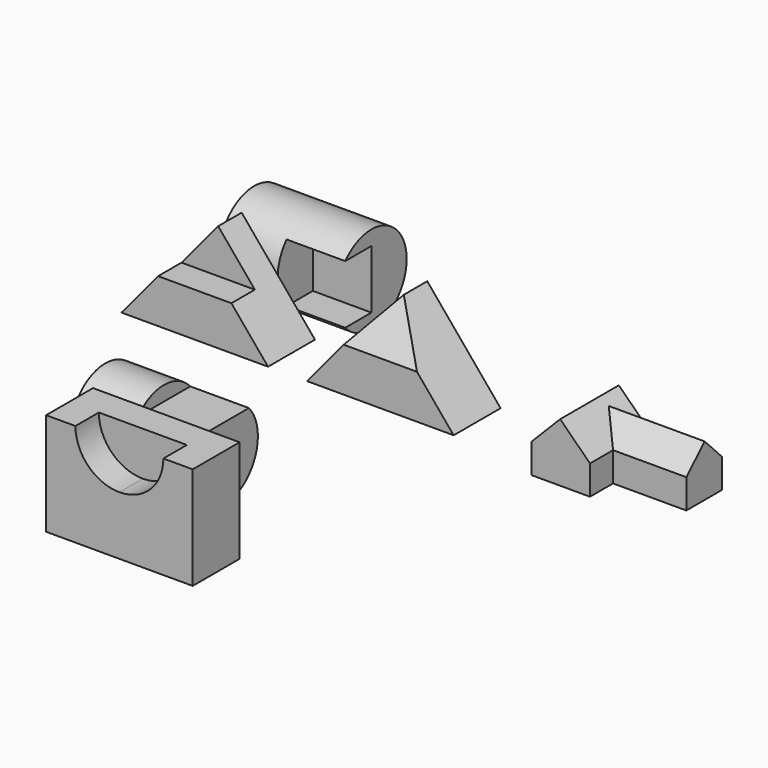
from build123d import *

# Parameters (mm, degrees)
F1_DEPTH  = 101.6
F3_DEPTH  = 50.8
F5_DEPTH  = 50.8
F8_DEPTH  = 254
F10_DEPTH = 101.6
F12_DEPTH = 127
F13_W     = 77.0500511372
F13_H     = 50.8
F14_DEPTH = 127
F17_DEPTH = 203.2
F20_DEPTH = 101.6
F22_DEPTH = 203.2
F24_DEPTH = 101.6
F25_W     = 101.6
F25_H     = 177.8
F26_DEPTH = 254
F28_DEPTH = 50.8


# Not quite as in the source:
# - a feature of the source that left no trace in its solid (it failed there, or was rolled back) is left out


with BuildPart() as f1:
    # F0 (on Front) → F1 (new body)
    with BuildSketch(Plane.XZ):
        Polygon((63.5, 76.2), (0, 0), (254, 0), (190.5, 76.2), align=None)
        Polygon((127, 152.4), (63.5, 76.2), (190.5, 76.2), align=None)
    extrude(amount=F1_DEPTH)

    # F2 (on face) → F3 (join)
    with BuildSketch(Plane.XZ.offset(101.6)):
        Polygon((127, 152.4), (63.5, 76.2), (190.5, 76.2), align=None)
    extrude(amount=-F3_DEPTH)

    # F4 (on face) → F5 (cut)
    with BuildSketch(Plane.XZ.offset(101.6)):
        Polygon((127, 152.4), (63.5, 76.2), (190.5, 76.2), align=None)
    extrude(amount=-F5_DEPTH, mode=Mode.SUBTRACT)


with BuildPart() as f8:
    # F7 (on offset) → F8 (new body)
    with BuildSketch(Plane.YZ.offset(321.564)):
        Polygon((-101.6, 0), (0, 0), (0, 152.4), (-50.8, 152.4), (-101.6, 76.2), align=None)
    extrude(amount=F8_DEPTH)

    # F9 (on face) → F10 (cut)
    with BuildSketch(Plane.XZ.offset(101.6)):
        Polygon((321.564, 76.2), (385.064, 76.2), (448.564, 152.4), (321.564, 152.4), align=None)
        Polygon((321.564, 76.2), (321.564, 0), (385.064, 76.2), align=None)
        Polygon((512.064, 76.2), (575.564, 0), (575.564, 76.2), align=None)
        Polygon((448.564, 152.4), (512.064, 76.2), (575.564, 76.2), (575.564, 152.4), align=None)
    extrude(amount=-F10_DEPTH, mode=Mode.SUBTRACT)


with BuildPart() as f12:
    # F11 (on Front) → F12 (new body)
    with BuildSketch(Plane.XZ):
        Polygon((730.4162154386, 50.8), (730.4162154386, 0), (781.2162154386, 0), (780.4500848747, 101.6), align=None)
        Polygon((780.4500848747, 101.6), (781.2162154386, 0), (832.0162154386, 0), (832.0162154386, 50.8), align=None)
    extrude(amount=F12_DEPTH)

    # F13 (on face) → F14 (join)
    with BuildSketch(Plane.YZ.offset(832.0162154386)):
        Polygon((-77.0500511372, 50.8), (0, 50.8), (-37.422735244, 89.3092527986), align=None)
        with Locations((-38.5250255686, 25.4)):
            Rectangle(F13_W, F13_H)
    extrude(amount=F14_DEPTH)

    # F13 (on face) → F15 (join, up to the next surface of F12)
    with BuildSketch(Plane.YZ.offset(832.0162154386)):
        Polygon((-77.0500511372, 50.8), (0, 50.8), (-37.422735244, 89.3092527986), align=None)
    extrude(until=Until.NEXT, dir=(-1, 0, 0))


with BuildPart() as f17:
    # F16 (on Right) → F17 (new body)
    with BuildSketch(Plane.YZ):
        with BuildLine():
            ThreePointArc((-136.3018900156, -215.5146067858), (-82.4203532892, -193.1961435122), (-60.1018900156, -139.3146067858))
            ThreePointArc((-60.1018900156, -139.3146067858), (-65.0951570451, -112.1845279125), (-79.4205561487, -88.6100324604))
            Line((-79.4205561487, -88.6100324604), (-140.1142077817, -88.6100324604))
            Line((-140.1142077817, -88.6100324604), (-193.1832238825, -88.6100324604))
            ThreePointArc((-193.1832238825, -88.6100324604), (-205.8365165106, -170.4815077899), (-136.3018900156, -215.5146067858))
        make_face()
        with BuildLine():
            Line((-140.1142077817, -88.6100324604), (-79.4205561487, -88.6100324604))
            ThreePointArc((-79.4205561487, -88.6100324604), (-136.3018900156, -63.1146067858), (-193.1832238825, -88.6100324604))
            Line((-193.1832238825, -88.6100324604), (-140.1142077817, -88.6100324604))
        make_face()
    extrude(amount=F17_DEPTH)

    # F18 (on face) → F20 (cut)
    with BuildSketch(Plane.YZ.offset(203.2)):
        with BuildLine():
            Line((-193.0983693738, -88.5150011523), (-136.5470457015, -88.5150011523))
            Line((-136.5470457015, -88.5150011523), (-79.5054106574, -88.5150011523))
            ThreePointArc((-79.5054106574, -88.5150011523), (-136.3018900156, -63.1146067858), (-193.0983693738, -88.5150011523))
        make_face()
    extrude(amount=-F20_DEPTH, mode=Mode.SUBTRACT)


with BuildPart() as f22:
    # F21 (on Right) → F22 (new body)
    with BuildSketch(Plane.YZ):
        with BuildLine():
            ThreePointArc((185.844445633, 76.2), (131.9629089065, -53.8815367264), (262.044445633, 0))
            ThreePointArc((262.044445633, 0), (239.7259823594, 53.8815367264), (185.844445633, 76.2))
        make_face()
    extrude(amount=F22_DEPTH)

    # F23 (on face) → F24 (cut)
    with BuildSketch(Plane.YZ.offset(203.2)):
        with BuildLine():
            ThreePointArc((129.0483190045, 50.8), (114.66051188, 27.1898432407), (109.644445633, 0))
            Line((109.644445633, 0), (185.844445633, 0))
            Line((185.844445633, 0), (185.844445633, 50.8))
            Line((185.844445633, 50.8), (129.0483190045, 50.8))
        make_face()
        with BuildLine():
            Line((185.844445633, 0), (109.644445633, 0))
            ThreePointArc((109.644445633, 0), (114.66051188, -27.1898432407), (129.0483190045, -50.8))
            Line((129.0483190045, -50.8), (185.844445633, -50.8))
            Line((185.844445633, -50.8), (185.844445633, 0))
        make_face()
    extrude(amount=-F24_DEPTH, mode=Mode.SUBTRACT)


with BuildPart() as f26:
    # F25 (on offset) → F26 (new body)
    with BuildSketch(Plane.YZ.offset(321.564)):
        with Locations((-615.9271565277, 88.9)):
            Rectangle(F25_W, F25_H)
    extrude(amount=F26_DEPTH)

    # F27 (on face) → F28 (cut)
    with BuildSketch(Plane.XZ.offset(666.7271565277)):
        with BuildLine():
            Line((448.564, 177.8), (448.564, 101.6))
            ThreePointArc((448.564, 101.6), (502.4455367264, 123.9184632736), (524.764, 177.8))
            Line((524.764, 177.8), (448.564, 177.8))
        make_face()
        with BuildLine():
            Line((448.564, 177.8), (372.364, 177.8))
            ThreePointArc((372.364, 177.8), (394.6824632736, 123.9184632736), (448.564, 101.6))
            Line((448.564, 101.6), (448.564, 177.8))
        make_face()
    extrude(amount=-F28_DEPTH, mode=Mode.SUBTRACT)


solid = Compound([f1.part, f8.part, f12.part, f17.part, f22.part, f26.part])
